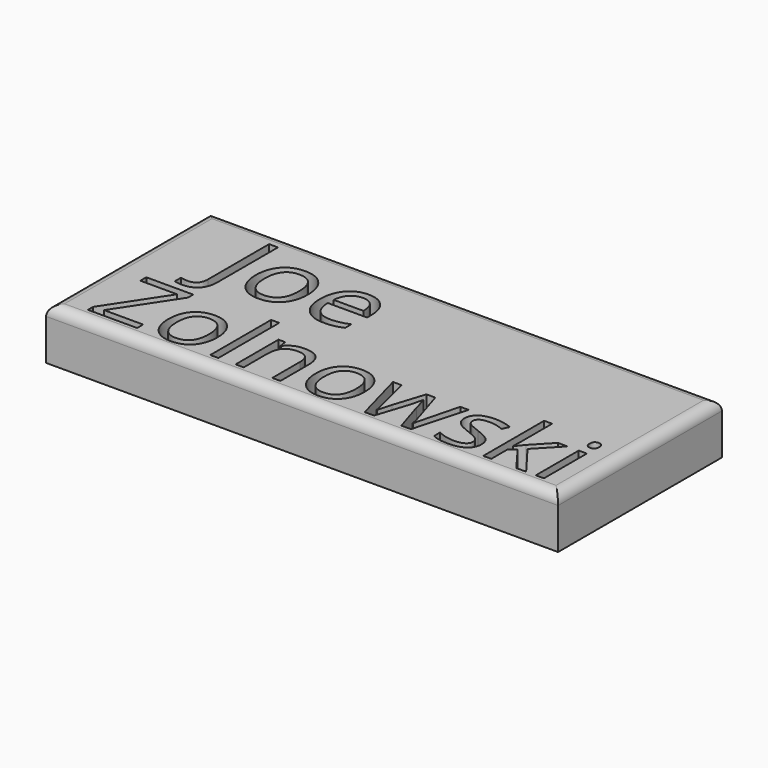
from build123d import *

# Parameters (mm, degrees)
F0_W           = 100
F0_H           = 40
F1_DEPTH       = 10
F2_TEXT_SIZE   = 20.8333333333
F2_TEXT_SIZE_2 = 19.5645528345
F3_DEPTH       = 5
F4_R           = 2
F5_TEXT_SIZE   = 9.8200887723
F6_DEPTH       = 3


# Not quite as in the source:
# - Text() gives the source's letters only with a copy of the font that has no kerning and outlines rounded to 1/6400 em; it was checked with that copy


with BuildPart() as f1:
    # F0 (on Top) → F1 (new body)
    with BuildSketch(Plane.XY):
        Rectangle(F0_W, F0_H)
    extrude(amount=F1_DEPTH)

    # F2 (on face) → F3 (cut)
    with BuildSketch(Plane.XY.offset(10)):
        with Locations((-37.8872093745, 2.0184680464)):
            Text('Joe', F2_TEXT_SIZE, font='Open Sans', text_align=(TextAlign.LEFT, TextAlign.BOTTOM))
        with Locations((-44.7487451136, -17.3233905468)):
            Text('Zolnowski', F2_TEXT_SIZE_2, font='Open Sans', text_align=(TextAlign.LEFT, TextAlign.BOTTOM))
    extrude(amount=-F3_DEPTH, mode=Mode.SUBTRACT)

    # F4
    f4_edges = [f1.edges().sort_by_distance(p)[0] for p in [
        (0, 20, 10),
        (-50, 0, 10),
        (0, -20, 10),
        (50, 0, 10),
    ]]
    fillet(f4_edges, radius=F4_R)

    # F5 (on face) → F6 (cut)
    with BuildSketch(Plane(origin=(0, 0, 0), x_dir=(1, 0, 0), z_dir=(0, 0, -1))):
        with Locations(Location((37.1471572239, -1.6064574507), (0, 0, 180))):
            Text('Good luck', F5_TEXT_SIZE, font='Open Sans', text_align=(TextAlign.LEFT, TextAlign.BOTTOM))
        with Locations(Location((37.1471572239, 11.7488632796), (0, 0, 180))):
            Text('your friend, Stan', F5_TEXT_SIZE, font='Open Sans', text_align=(TextAlign.LEFT, TextAlign.BOTTOM))
    extrude(amount=-F6_DEPTH, mode=Mode.SUBTRACT)


solid = f1.part
